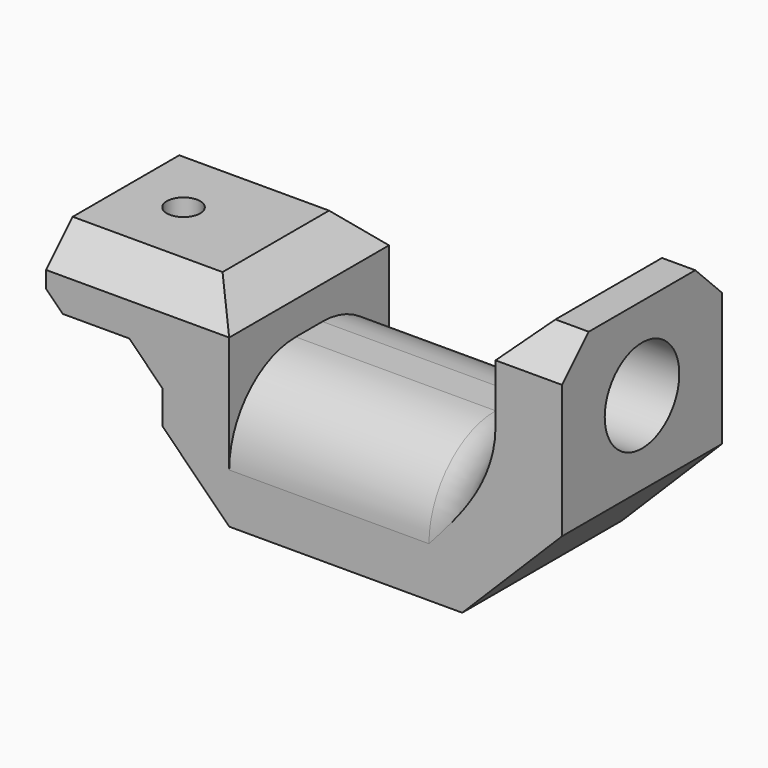
from build123d import *

# Parameters (mm, degrees)
F0_W         = 80
F0_H         = 40
F1_DEPTH     = 60
F2_R         = 25
F4_D         = 10
F5_T1_DEPTH  = 10
F5_T6_ANGLE  = 204.6375913899
F5_T12_ANGLE = 204.6375913899
F6_SIZE      = 10
F7_SIZE      = 30
F8_SIZE      = 20
F10_D        = 28
F10_DEPTH    = 50
F10_TIP      = 8.4120486664
F11_SIZE     = 5
F12_SIZE     = 10


# Not quite as in the source:
# - a fillet or chamfer that OpenCascade refuses, or shapes differently, is made with other operations: its cross-section is extruded or revolved along the edge and cut away or added


with BuildPart() as f1:
    # F0 (on Front) → F1 (new body)
    with BuildSketch(Plane.XZ):
        Rectangle(F0_W, F0_H)
        Polygon((40, 60), (40, 20), (40, -20), (60, -20), (60, 60), align=None)
        Polygon((-40, -20), (-40, 20), (-40, 40), (-60, 40), (-60, 20), (-60, -20), align=None)
        Polygon((-60, 20), (-60, 40), (-80, 40), (-95, 40), (-95, 20), (-80, 20), align=None)
    extrude(amount=F1_DEPTH)

    # F2
    f2_edges = [f1.edges().sort_by_distance(p)[0] for p in [
        (0, -60, 20),
        (0, 0, 20),
    ]]
    fillet(f2_edges, radius=F2_R)

    # F4 (through all)
    with Locations(Plane.XY.offset(40)):
        with Locations((-77.7127879113, -30)):
            Hole(F4_D / 2)

    # F5: fillet of radius 20 on 1 edges, made by hand

    # F5_s2 → F5_t1 (join)
    with BuildSketch(Plane.XZ.offset(25)):
        with BuildLine():
            ThreePointArc((20, 20), (34.1421356237, 25.8578643763), (40, 40))
            Line((40, 40), (40, 20))
            Line((40, 20), (20, 20))
        make_face()
    extrude(amount=F5_T1_DEPTH)


with BuildPart() as f5_tool4:
    # F5_s5 → F5_t6 (revolve)
    with BuildSketch(Plane.XZ.offset(25)):
        with BuildLine():
            ThreePointArc((20, 20), (34.1421356237, 25.8578643763), (40, 40))
            Line((40, 40), (40, 20))
            Line((40, 20), (20, 20))
        make_face()
    revolve(axis=Axis((40, -25, -5), (-1, 0, 0)), revolution_arc=F5_T6_ANGLE)

    split(bisect_by=Plane.XZ, keep=Keep.TOP)

    split(bisect_by=Plane.XY.offset(-20), keep=Keep.TOP)


with BuildPart() as f1_1:
    add(f1.part)

    # F5_t3: union F5_tool4
    add(f5_tool4.part)


with BuildPart() as f5_tool10:
    # F5_s11 → F5_t12 (revolve)
    with BuildSketch(Plane.XZ.offset(35)):
        with BuildLine():
            ThreePointArc((20, 20), (34.1421356237, 25.8578643763), (40, 40))
            Line((40, 40), (40, 20))
            Line((40, 20), (20, 20))
        make_face()
    revolve(axis=Axis((40, -35, -5), (1, 0, 0)), revolution_arc=F5_T12_ANGLE)

    split(bisect_by=Plane.XY.offset(-20), keep=Keep.TOP)

    split(bisect_by=Plane.XZ.offset(60), keep=Keep.BOTTOM)


with BuildPart() as f1_2:
    add(f1_1.part)

    # F5_t9: union F5_tool10
    add(f5_tool10.part)

    # F6
    f6_edges = [f1_2.edges().sort_by_distance(p)[0] for p in [
        (-67.5, -60, 40),
        (-67.5, 0, 40),
        (50, -60, 60),
        (50, 0, 60),
        (-40, -30, 40),
        (40, -30, 60),
    ]]
    chamfer(f6_edges, length=F6_SIZE)

    # F7
    f7_edges = [f1_2.edges().sort_by_distance(p)[0] for p in [
        (60, -30, -20),
    ]]
    chamfer(f7_edges, length=F7_SIZE)

    # F8
    f8_edges = [f1_2.edges().sort_by_distance(p)[0] for p in [
        (-60, -30, -20),
    ]]
    chamfer(f8_edges, length=F8_SIZE)

    # F10
    with Locations(Plane.YZ.offset(60)):
        with Locations((-30, 35)):
            Hole(F10_D / 2, depth=F10_DEPTH)
            with Locations((0, 0, -(F10_DEPTH + F10_TIP / 2))):  # 118° drill point
                Cone(0, F10_D / 2, F10_TIP, mode=Mode.SUBTRACT)

    # F11
    f11_edges = [f1_2.edges().sort_by_distance(p)[0] for p in [
        (-95, -30, 20),
    ]]
    chamfer(f11_edges, length=F11_SIZE)

    # F12
    f12_edges = [f1_2.edges().sort_by_distance(p)[0] for p in [
        (-60, -30, 20),
    ]]
    chamfer(f12_edges, length=F12_SIZE)


solid = f1_2.part
